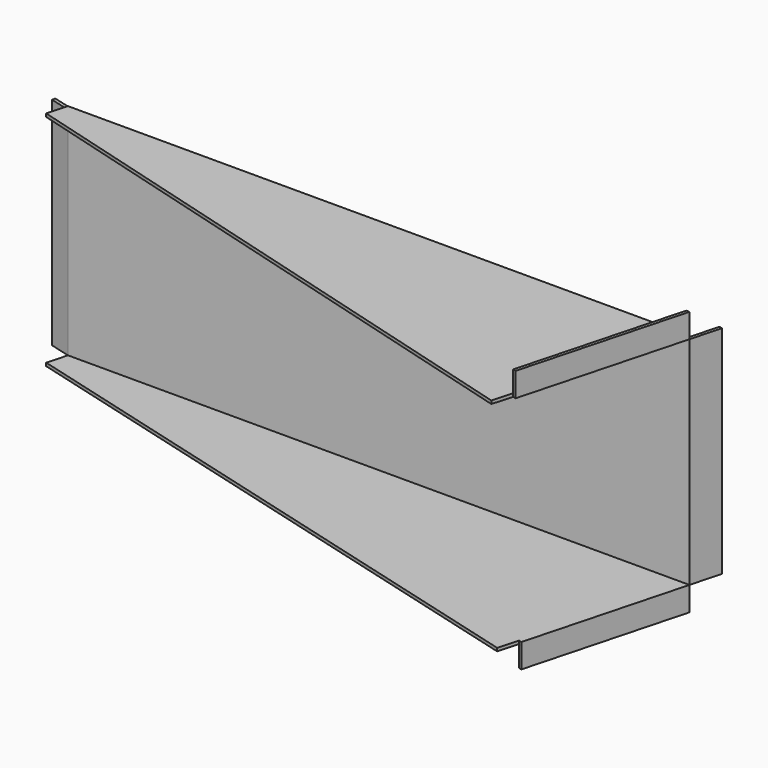
from build123d import *

# Parameters (mm, degrees)
F0_W      = 580
F0_H      = 206
F1_DEPTH  = 3
F3_DEPTH  = 206
F4_W      = 3.1058285412
F4_H      = 206
F5_DEPTH  = 20
F6_DEPTH  = 206
F7_W      = 3
F7_H      = 206
F8_DEPTH  = 30
F9_DEPTH  = 3
F11_DEPTH = 3
F13_DEPTH = 20
F15_DEPTH = 20
F16_W     = 568.8317526069
F16_H     = 3
F17_DEPTH = 20
F18_W     = 568.8756012417
F18_H     = 3
F19_DEPTH = 20


# Not quite as in the source:
# - a feature names something its author has since deleted; it is built from what else it names


with BuildPart() as f1:
    # F0 (on Front) → F1 (new body)
    with BuildSketch(Plane.XZ):
        Rectangle(F0_W, F0_H)
    extrude(amount=F1_DEPTH)

    # F2 (on face) → F3 (join)
    with BuildSketch(Plane.XY.offset(103)):
        Polygon((-290, -3), (-290, 0), (-290.8038475773, -3), align=None)
    extrude(amount=-F3_DEPTH)

    # F4 (on face) → F5 (join)
    with BuildSketch(Plane(origin=(-270.5736835487, 72.5, 0), x_dir=(-0.2588190451, -0.9659258263, 0), z_dir=(-0.9659258263, 0.2588190451, 0))):
        with Locations((76.6104373503, 0)):
            Rectangle(F4_W, F4_H)
    extrude(amount=F5_DEPTH)

    # F2 (on face) → F6 (join)
    with BuildSketch(Plane.XY.offset(103)):
        Polygon((301.1961524227, -3), (290, 0), (290, -3), align=None)
    extrude(amount=-F6_DEPTH)

    # F7 (on face) → F8 (join)
    with BuildSketch(Plane(origin=(19.4263164513, 72.5, 0), x_dir=(-0.9659258263, 0.2588190451, 0), z_dir=(0.2588190451, 0.9659258263, 0))):
        with Locations((-290.2095995393, 0)):
            Rectangle(F7_W, F7_H)
    extrude(amount=F8_DEPTH)



with BuildPart() as f9:
    # F2 (on face) → F9 (new body)
    with BuildSketch(Plane.XY.offset(103)):
        Polygon((-290, -3), (-290.8038475773, -3), (259.6317745839, -158.1203698794), (301.1961524227, -3), (290, -3), align=None)
    extrude(amount=F9_DEPTH)

    # F14 (on face) → F15 (join)
    with BuildSketch(Plane.XY.offset(106)):
        Polygon((256.7442464871, -157.3066245323), (259.6317745839, -158.1203698794), (301.1961524227, -3), (298.0903238817, -3), align=None)
    extrude(amount=F15_DEPTH)


with BuildPart() as f11:
    # F10 (on face) → F11 (new body)
    with BuildSketch(Plane(origin=(0, 0, -103), x_dir=(1, 0, 0), z_dir=(0, 0, -1))):
        Polygon((261.0098994174, 152.9771379815), (-290.8038475773, 3), (301.1961524227, 3), align=None)
    extrude(amount=F11_DEPTH)

    # F12 (on face) → F13 (join)
    with BuildSketch(Plane(origin=(0, 0, -106), x_dir=(1, 0, 0), z_dir=(0, 0, -1))):
        Polygon((301.1961524227, 3), (261.0098994174, 152.9771379815), (258.1149198479, 152.1903131648), (298.0903240127, 3), align=None)
    extrude(amount=F13_DEPTH)


with BuildPart() as f1_1:
    add(f1.part)

    add(f11.part)  # F17 merges F11
    # F16 (on face) → F17 (join)
    with BuildSketch(Plane(origin=(-20.7631374105, -76.3942078643, 0), x_dir=(0.9649931898, -0.2622749389, 0), z_dir=(-0.2622749389, -0.9649931898, 0))):
        with Locations((4.5789686315, -104.5)):
            Rectangle(F16_W, F16_H)
    extrude(amount=F17_DEPTH)


    add(f9.part)  # F19 merges F9
    # F18 (on face) → F19 (join)
    with BuildSketch(Plane(origin=(-22.1793403036, -78.7021007532, 0), x_dir=(0.9625093656, -0.271248449, 0), z_dir=(-0.271248449, -0.9625093656, 0))):
        with Locations((5.3501191182, 104.5)):
            Rectangle(F18_W, F18_H)
    extrude(amount=F19_DEPTH)


solid = f1_1.part
